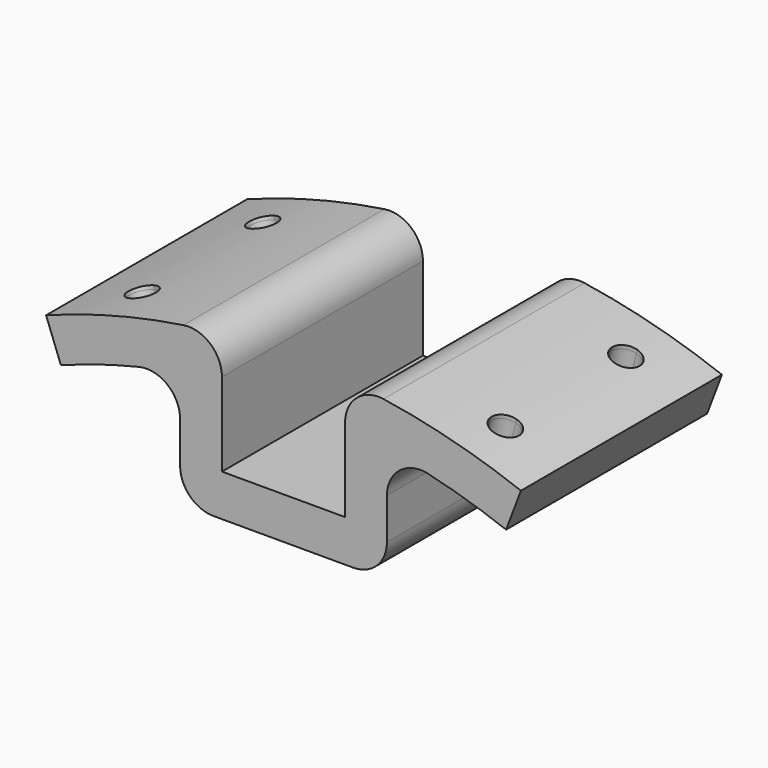
from build123d import *

# Parameters (mm, degrees)
F1_DEPTH = 38.1
F2_R     = 5.08
F7_DEPTH = 12.7
F8_DEPTH = 12.7


# Not quite as in the source:
# - a pattern or mirror of a feature is missing from the dataset's text; its kind, count and spacing are read off the source's solid


with BuildPart() as f1:
    # F0 (on Front) → F1 (new body)
    with BuildSketch(Plane.XZ):
        with BuildLine():
            Line((-9.3345, 82.804), (-9.3345, 101.1702876825))
            ThreePointArc((-9.3345, 101.1702876825), (-22.880190841, 98.9901857109), (-36.0086465439, 95.0049334197))
            Line((-36.0086465439, 95.0049334197), (-33.7581061349, 89.067125081))
            ThreePointArc((-33.7581061349, 89.067125081), (-24.8415554365, 91.9535731959), (-15.6845, 93.9497682794))
            Line((-15.6845, 93.9497682794), (-15.6845, 76.454))
            Line((-15.6845, 76.454), (15.6845, 76.454))
            Line((15.6845, 76.454), (15.6845, 93.9497682794))
            ThreePointArc((15.6845, 93.9497682794), (24.8415554365, 91.9535731959), (33.7581061349, 89.067125081))
            Line((33.7581061349, 89.067125081), (36.0086465439, 95.0049334197))
            ThreePointArc((36.0086465439, 95.0049334197), (22.880190841, 98.9901857109), (9.3345, 101.1702876825))
            Line((9.3345, 101.1702876825), (9.3345, 82.804))
            Line((9.3345, 82.804), (-9.3345, 82.804))
        make_face()
    extrude(amount=F1_DEPTH)

    # F2
    f2_edges = [f1.edges().sort_by_distance(p)[0] for p in [
        (-9.3345, -19.05, 101.170288),
        (9.3345, -19.05, 101.170288),
        (15.6845, -19.05, 93.949768),
        (-15.6845, -19.05, 93.949768),
        (15.6845, -19.05, 76.454),
        (-15.6845, -19.05, 76.454),
    ]]
    fillet(f2_edges, radius=F2_R)

    # F4 (on face) → F7 (cut, symmetric)
    with BuildSketch(Plane(origin=(-25.5909022193, 0, 97.7327744919), x_dir=(0.9673862364, 0, 0.2533058814), z_dir=(0.2533058814, 0, -0.9673862364))):
        with BuildLine():
            Line((-1.8789606614, 5.461), (-1.8789606614, 9.779))
            ThreePointArc((-1.8789606614, 9.779), (-4.0379606614, 7.62), (-1.8789606614, 5.461))
        make_face()
    extrude(amount=F7_DEPTH, both=True, mode=Mode.SUBTRACT)

    # F4 (on face) → F8 (cut, symmetric)
    with BuildSketch(Plane(origin=(-25.5909022193, 0, 97.7327744919), x_dir=(0.9673862364, 0, 0.2533058814), z_dir=(0.2533058814, 0, -0.9673862364))):
        with BuildLine():
            ThreePointArc((-1.8789606614, 32.639), (-4.0379606614, 30.48), (-1.8789606614, 28.321))
            Line((-1.8789606614, 28.321), (-1.8789606614, 30.48))
            Line((-1.8789606614, 30.48), (-1.8789606614, 32.639))
        make_face()
        with BuildLine():
            Line((-1.8789606614, 30.48), (-1.8789606614, 28.321))
            ThreePointArc((-1.8789606614, 28.321), (-0.3523171208, 28.9533564594), (0.2800393386, 30.48))
            ThreePointArc((0.2800393386, 30.48), (-0.3523171208, 32.0066435406), (-1.8789606614, 32.639))
            Line((-1.8789606614, 32.639), (-1.8789606614, 30.48))
        make_face()
        with BuildLine():
            ThreePointArc((-1.8789606614, 5.461), (-0.3523171208, 6.0933564594), (0.2800393386, 7.62))
            ThreePointArc((0.2800393386, 7.62), (-0.3523171208, 9.1466435406), (-1.8789606614, 9.779))
            Line((-1.8789606614, 9.779), (-1.8789606614, 5.461))
        make_face()
        with BuildLine():
            Line((-1.8789606614, 5.461), (-1.8789606614, 9.779))
            ThreePointArc((-1.8789606614, 9.779), (-4.0379606614, 7.62), (-1.8789606614, 5.461))
        make_face()
    f8 = extrude(amount=F8_DEPTH, both=True, mode=Mode.SUBTRACT)

    # F8_copies: F8 across plane
    add(f8.mirror(Plane(origin=(6e-06, 0, 0), x_dir=(0, 0, 1), z_dir=(1, 0, 0))), mode=Mode.SUBTRACT)


solid = f1.part
